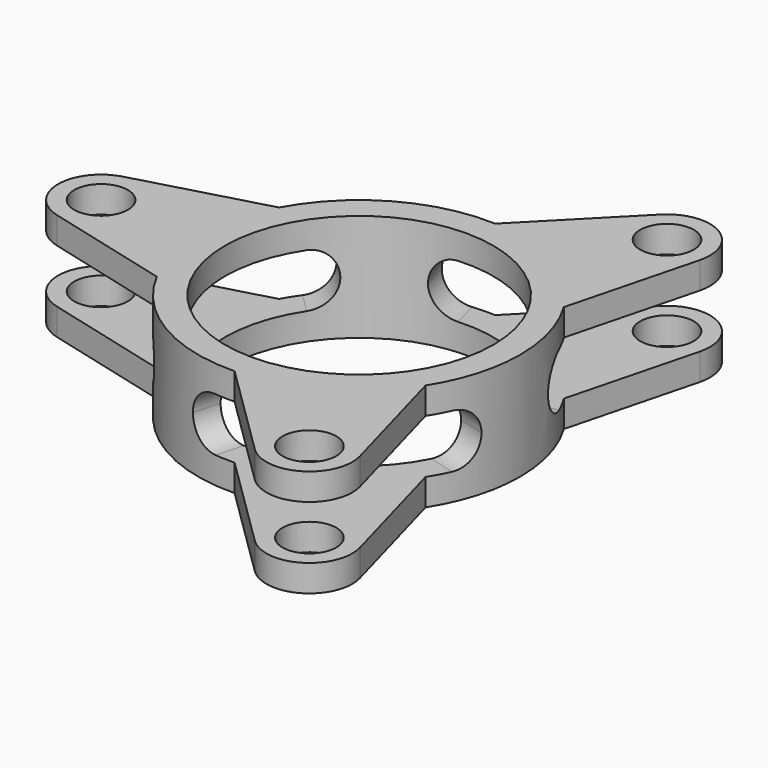
from build123d import *

# Parameters (mm, degrees)
F0_R          = 25
F0_R_2        = 5
F1_DEPTH      = 10
F1_DEPTH_BACK = 10
F2_W          = 70
F2_H          = 10
F3_ANGLE_BACK = 45
F3_ANGLE      = 90
F4_COUNT      = 3
F4_ANGLE      = 240
F6_R          = 4.99999


# Not quite as in the source:
# - a fillet or chamfer is up to 0.001 mm smaller than in the source, because OpenCascade refuses the exact size


with BuildPart() as f1:
    # F0 (on Top) → F1 (new body, two sides)
    with BuildSketch(Plane.XY) as f1_sk:
        with BuildLine():
            ThreePointArc((25.282899435, -16.1485292259), (28.7965881924, -8.4116888004), (30, 0))
            ThreePointArc((30, 0), (28.8728814443, 8.1459632398), (25.5762188598, 15.6798287247))
            ThreePointArc((25.5762188598, 15.6798287247), (15.2387828621, 25.8414298537), (1.3435868258, 29.969897805))
            ThreePointArc((1.3435868258, 29.969897805), (-14.7599432924, 26.1178880081), (-26.3672394325, 14.3097409029))
            ThreePointArc((-26.3672394325, 14.3097409029), (-29.9987261544, 0.2764581545), (-26.6264862609, -13.8213685791))
            ThreePointArc((-26.6264862609, -13.8213685791), (-15.2387828621, -25.8414298537), (0.7910205727, -29.9895696277))
            ThreePointArc((0.7910205727, -29.9895696277), (14.7599432924, -26.1178880081), (25.282899435, -16.1485292259))
        make_face()
        Circle(F0_R, mode=Mode.SUBTRACT)
        with BuildLine():
            ThreePointArc((1.3435868258, 29.969897805), (15.2387828621, 25.8414298537), (25.5762188598, 15.6798287247))
            Line((25.5762188598, 15.6798287247), (31.7810181804, 39.6262733222))
            ThreePointArc((31.7810181804, 39.6262733222), (27.9793762729, 48.5939196708), (18.3333577354, 47.2428132348))
            Line((18.3333577354, 47.2428132348), (1.3435868258, 29.969897805))
        make_face()
        with Locations((24.0367650986, 41.6328984003)):
            Circle(F0_R_2, mode=Mode.SUBTRACT)
        with BuildLine():
            Line((31.7467975399, -39.4985601529), (25.282899435, -16.1485292259))
            ThreePointArc((25.282899435, -16.1485292259), (14.7599432924, -26.1178880081), (0.7910205727, -29.9895696277))
            Line((0.7910205727, -29.9895696277), (18.4268502641, -47.3363057635))
            ThreePointArc((18.4268502641, -47.3363057635), (28.0938807679, -48.5278104698), (31.7467975399, -39.4985601529))
        make_face()
        with Locations((24.0367650986, -41.6328984003)):
            Circle(F0_R_2, mode=Mode.SUBTRACT)
        with BuildLine():
            ThreePointArc((-26.6264862609, -13.8213685791), (-29.9987261544, 0.2764581545), (-26.3672394325, 14.3097409029))
            Line((-26.3672394325, 14.3097409029), (-50.2078684445, 7.7100324413))
            ThreePointArc((-50.2078684445, 7.7100324413), (-56.0732570408, -0.066109201), (-50.0801552753, -7.7442530819))
            Line((-50.0801552753, -7.7442530819), (-26.6264862609, -13.8213685791))
        make_face()
        with Locations((-48.0735301971, 0)):
            Circle(F0_R_2, mode=Mode.SUBTRACT)
    extrude(amount=F1_DEPTH)
    extrude(f1_sk.sketch, amount=-F1_DEPTH_BACK)


with BuildPart() as f3:
    # F2 (on Front) → F3 (revolve)
    with BuildSketch(Plane.XZ, mode=Mode.PRIVATE) as f3_sk:
        with Locations((-34.9688172646, 0)):
            Rectangle(F2_W, F2_H)
    revolve(f3_sk.sketch.rotate(Axis((0.0311827354, 0, 0), (0, 0, -1)), -F3_ANGLE_BACK), axis=Axis((0.0311827354, 0, 0), (0, 0, -1)), revolution_arc=F3_ANGLE)


with BuildPart() as f4_1:
    # F4: instance of F3
    add(f3.part.rotate(Axis((0, 0, 10), (0, 0, -1)), 1 * F4_ANGLE / (F4_COUNT - 1)))


with BuildPart() as f4_2:
    # F4: instance of F3
    add(f3.part.rotate(Axis((0, 0, 10), (0, 0, -1)), 2 * F4_ANGLE / (F4_COUNT - 1)))


with BuildPart() as f1_1:
    add(f1.part)

    # F5: cut F3, F4_1, F4_2
    add(f3.part, mode=Mode.SUBTRACT)
    add(f4_1.part, mode=Mode.SUBTRACT)
    add(f4_2.part, mode=Mode.SUBTRACT)

    # F6 (radius 5 in the source; OpenCascade refuses exactly that, so slightly less here)
    f6_edges = [f1_1.edges().sort_by_distance(p)[0] for p in [
        (26.568658, 7.096223, 5),
        (26.568658, 7.096223, -5),
        (26.568658, -7.096223, -5),
        (26.568658, -7.096223, 5),
        (-7.13882, -26.557245, 5),
        (-7.13882, -26.557245, -5),
        (-19.429839, 19.461022, -5),
        (-7.13882, 26.557245, -5),
        (-19.429839, 19.461022, 5),
        (-7.13882, 26.557245, 5),
        (-19.429839, -19.461022, -5),
        (-19.429839, -19.461022, 5),
    ]]
    fillet(f6_edges, radius=F6_R)


solid = f1_1.part
